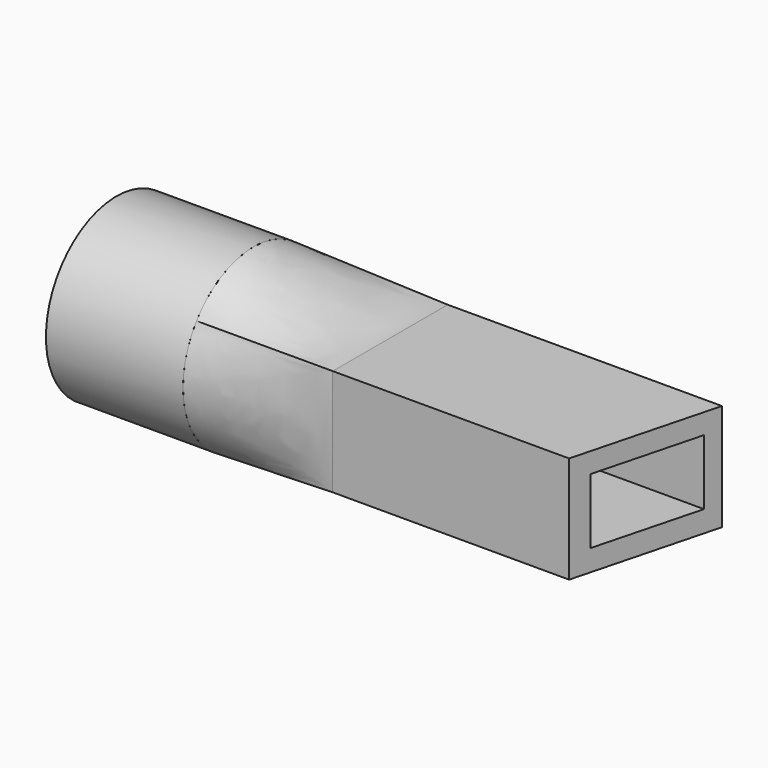
from build123d import *

# Parameters (mm, degrees)
F0_R      = 49.0134805441
F1_DEPTH  = 76.2
F3_W      = 79.9200758338
F3_H      = 59.3156740069
F5_DEPTH  = 152.4
F7_DEPTH  = 59.3156740069
F9_W      = 59.3156721443
F9_H      = 36.2137816846
F10_DEPTH = 152.4
F11_R     = 27.8477837619
F12_DEPTH = 76.2


# Not quite as in the source:
# - a feature of the source that left no trace in its solid (it failed there, or was rolled back) is left out
# - the arcs of a loft's sections are written as splines that run evenly, so that the points pair up as in the source's solid


with BuildPart() as f1:
    # F0 (on Right) → F1 (new body)
    with BuildSketch(Plane.YZ):
        Circle(F0_R)
    extrude(amount=F1_DEPTH)

    # F11 (on face) → F12 (cut, through all)
    with BuildSketch(Plane(origin=(0, 0, 0), x_dir=(0, -1, 0), z_dir=(-1, 0, 0))):
        Circle(F11_R)
    extrude(amount=-F12_DEPTH, mode=Mode.SUBTRACT)


with BuildPart() as f4:
    # F1_face (on face) → F4 section 0
    with BuildSketch(Plane.YZ.offset(76.2)):
        with BuildLine():
            add(Edge.make_bspline(
                [(-39.6123992828, 28.8648419033), (-41.5015987676, 26.272216433), (-43.1354065314, 23.4935897628), (-45.8296123485, 17.6708428932), (-46.8899437823, 14.6268666727), (-48.3964196283, 8.3903887711), (-48.8425267899, 5.1980412992), (-49.1033796429, -1.2125032862), (-48.9181188841, -4.4305418863), (-47.9233243152, -10.7687995221), (-47.1138151033, -13.8888618319), (-44.9016025099, -19.9112568317), (-43.4989538297, -22.8134406061), (-40.1543373011, -28.2885357075), (-38.212452155, -30.8613116519), (-33.8639634288, -35.5787020205), (-31.4574673737, -37.723199798), (-28.8648419033, -39.6123992828)],
                knots=[0, 0, 0, 0, 0.125, 0.125, 0.25, 0.25, 0.375, 0.375, 0.5, 0.5, 0.625, 0.625, 0.75, 0.75, 0.875, 0.875, 1, 1, 1, 1], degree=3))
            add(Edge.make_bspline(
                [(-28.8648419033, -39.6123992828), (-26.272216433, -41.5015987676), (-23.4935897628, -43.1354065314), (-17.6708428932, -45.8296123485), (-14.6268666727, -46.8899437823), (-8.3903887711, -48.3964196283), (-5.1980412992, -48.8425267899), (1.2125032862, -49.1033796429), (4.4305418863, -48.9181188841), (10.7687995221, -47.9233243152), (13.8888618319, -47.1138151033), (19.9112568317, -44.9016025099), (22.8134406061, -43.4989538297), (28.2885357075, -40.1543373011), (30.8613116519, -38.212452155), (35.5787020205, -33.8639634288), (37.723199798, -31.4574673737), (39.6123992828, -28.8648419033)],
                knots=[0, 0, 0, 0, 0.125, 0.125, 0.25, 0.25, 0.375, 0.375, 0.5, 0.5, 0.625, 0.625, 0.75, 0.75, 0.875, 0.875, 1, 1, 1, 1], degree=3))
            add(Edge.make_bspline(
                [(39.6123992828, -28.8648419033), (41.5015987676, -26.272216433), (43.1354065314, -23.4935897628), (45.8296123485, -17.6708428932), (46.8899437823, -14.6268666727), (48.3964196283, -8.3903887711), (48.8425267899, -5.1980412992), (49.1033796429, 1.2125032862), (48.9181188841, 4.4305418863), (47.9233243152, 10.7687995221), (47.1138151033, 13.8888618319), (44.9016025099, 19.9112568317), (43.4989538297, 22.8134406061), (40.1543373011, 28.2885357075), (38.212452155, 30.8613116519), (33.8639634288, 35.5787020205), (31.4574673737, 37.723199798), (28.8648419033, 39.6123992828)],
                knots=[0, 0, 0, 0, 0.125, 0.125, 0.25, 0.25, 0.375, 0.375, 0.5, 0.5, 0.625, 0.625, 0.75, 0.75, 0.875, 0.875, 1, 1, 1, 1], degree=3))
            add(Edge.make_bspline(
                [(28.8648419033, 39.6123992828), (26.272216433, 41.5015987676), (23.4935897628, 43.1354065314), (17.6708428932, 45.8296123485), (14.6268666727, 46.8899437823), (8.3903887711, 48.3964196283), (5.1980412992, 48.8425267899), (-1.2125032862, 49.1033796429), (-4.4305418863, 48.9181188841), (-10.7687995221, 47.9233243152), (-13.8888618319, 47.1138151033), (-19.9112568317, 44.9016025099), (-22.8134406061, 43.4989538297), (-28.2885357075, 40.1543373011), (-30.8613116519, 38.212452155), (-35.5787020205, 33.8639634288), (-37.723199798, 31.4574673737), (-39.6123992828, 28.8648419033)],
                knots=[0, 0, 0, 0, 0.125, 0.125, 0.25, 0.25, 0.375, 0.375, 0.5, 0.5, 0.625, 0.625, 0.75, 0.75, 0.875, 0.875, 1, 1, 1, 1], degree=3))
        make_face()
    # F3 (on offset) → F4 section 1
    with BuildSketch(Plane.YZ.offset(152.4)):
        with Locations((-0.3121942282, -0.3121867776)):
            Rectangle(F3_W, F3_H)
    loft(ruled=True)

    # F5 (add): a face of the model
    f5_faces = [f4.faces().sort_by_distance(p)[0] for p in [
        (152.4, -0.3121942282, -0.3121867776),
    ]]
    extrude(f5_faces, amount=F5_DEPTH)

    # F6 (on face) → F7 (cut, through all)
    with BuildSketch(Plane.XY.offset(29.3456502259)):
        Polygon((304.8, -40.2722321451), (304.8, 39.6478436887), (283.8114500046, -40.2722321451), align=None)
    extrude(amount=-F7_DEPTH, mode=Mode.SUBTRACT)

    # F9 (on offset) → F10 (cut)
    with BuildSketch(Plane.YZ.offset(304.8)):
        with Locations((0.6243688986, 3.7253e-06)):
            Rectangle(F9_W, F9_H)
    extrude(amount=-F10_DEPTH, mode=Mode.SUBTRACT)


solid = Compound([f1.part, f4.part])
